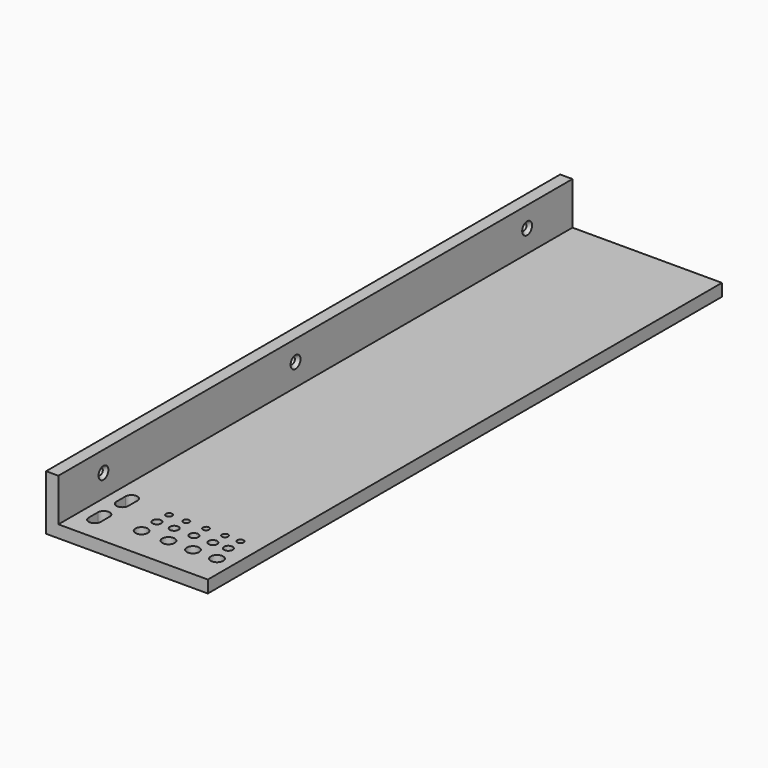
from build123d import *

# Parameters (mm, degrees)
F0_W            = 307.8816831112
F0_H            = 200.2553716302
F1_DEPTH        = 25.4
F2_W            = 307.8816831112
F2_H            = 25.4
F3_DEPTH        = 174.76264
F4_DEPTH        = 949.00905
F5_W            = 1324.0270616302
F5_H            = 25.4
F6_DEPTH        = 25.4
F7_W            = 25.4
F7_H            = 1324.0270616302
F8_DEPTH        = 88.17008
F10_D           = 12.7
F10_CSINK_D     = 25.4
F10_CSINK_ANGLE = 90
F12_D           = 12.7
F13_D           = 17.78
F14_D           = 25.4
F15_DEPTH       = 25.4


with BuildPart() as f1:
    # F0 (on Top) → F1 (new body)
    with BuildSketch(Plane.XY):
        with Locations((-0.1046210527, -15.8108584583)):
            Rectangle(F0_W, F0_H)
    extrude(amount=F1_DEPTH)

    # F2 (on face) → F3 (join)
    with BuildSketch(Plane(origin=(0, 84.3168273568, 0), x_dir=(-1, 0, 0), z_dir=(0, 1, 0))):
        with Locations((0.1046210527, 12.7)):
            Rectangle(F2_W, F2_H)
    extrude(amount=F3_DEPTH)

    # F4 (add): a face of the model
    f4_faces = [f1.faces().sort_by_distance(p)[0] for p in [
        (-0.1046210527, 259.0794673568, 12.7),
    ]]
    extrude(f4_faces, amount=F4_DEPTH)

    # F5 (on face) → F6 (join)
    with BuildSketch(Plane(origin=(-154.0454626083, 0, 0), x_dir=(0, -1, 0), z_dir=(-1, 0, 0))):
        with Locations((-546.0749865417, 12.7)):
            Rectangle(F5_W, F5_H)
    extrude(amount=F6_DEPTH)

    # F7 (on face) → F8 (join)
    with BuildSketch(Plane.XY.offset(25.4)):
        with Locations((-166.7454626083, 546.0749865417)):
            Rectangle(F7_W, F7_H)
    extrude(amount=F8_DEPTH)

    # F10 (through all)
    with Locations(Plane.YZ.offset(-154.0454626083)):
        with Locations((0, 71.7426463962), (494.805842638, 71.7426463962), (1091.2485173568, 71.7426463962)):
            CounterSinkHole(F10_D / 2, F10_CSINK_D / 2, counter_sink_angle=F10_CSINK_ANGLE)

    # F12 (through all)
    with Locations(Plane.XY.offset(25.4)):
        with Locations((-35.56, 21.0037976503), (0, 21.0037976503), (40.685325861, 21.0037976503), (79.7552913427, 21.0037976503), (111.532188952, 21.0037976503)):
            Hole(F12_D / 2)

    # F13 (through all)
    with Locations(Plane.XY.offset(25.4)):
        with Locations((-35.56, -10.2521730587), (0, -10.2521730587), (40.685325861, -10.2521730587), (79.7552913427, -10.2521730587), (111.532188952, -10.2521730587)):
            Hole(F13_D / 2)

    # F14 (through all)
    with Locations(Plane.XY.offset(25.4)):
        with Locations((-35.56, -49.8430728912), (19.8480077088, -49.8430728912), (70.3785046935, -49.8430728912), (119.8671087623, -49.8430728912)):
            Hole(F14_D / 2)

    # F11 (on face) → F15 (cut)
    with BuildSketch(Plane.XY.offset(25.4)):
        with BuildLine():
            Line((-130.6297034025, 27.7527463882), (-130.6297034025, 4.3339463882))
            ThreePointArc((-130.6297034025, 4.3339463882), (-118.4733323753, -7.822424639), (-106.3169613481, 4.3339463882))
            Line((-106.3169613481, 4.3339463882), (-106.3169613481, 27.7527463882))
            ThreePointArc((-106.3169613481, 27.7527463882), (-118.4733323753, 39.9091174154), (-130.6297034025, 27.7527463882))
        make_face()
        with BuildLine():
            ThreePointArc((-106.3169613481, -43.5644686222), (-118.4733323753, -31.408097595), (-130.6297034025, -43.5644686222))
            Line((-130.6297034025, -43.5644686222), (-130.6297034025, -63.3748397231))
            Line((-130.6297034025, -63.3748397231), (-130.6297034025, -66.9767335057))
            ThreePointArc((-130.6297034025, -66.9767335057), (-118.4733323753, -79.133104533), (-106.3169613481, -66.9767335057))
            Line((-106.3169613481, -66.9767335057), (-106.3169613481, -43.5644686222))
        make_face()
    extrude(amount=-F15_DEPTH, mode=Mode.SUBTRACT)


solid = f1.part
